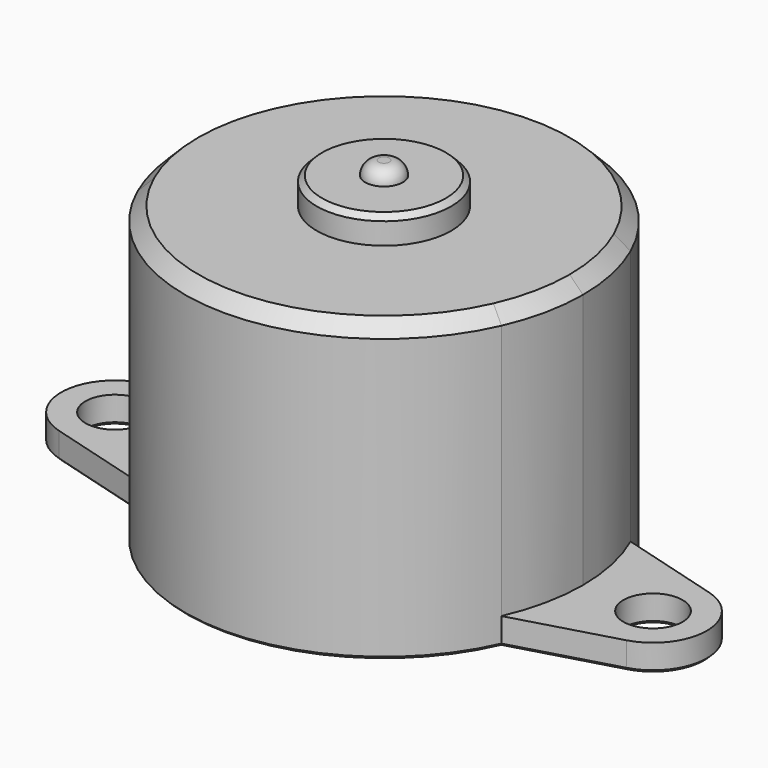
from build123d import *

# Parameters (mm, degrees)
F0_R     = 1.1
F1_DEPTH = 1
F3_DEPTH = 10
F4_R     = 2.5
F5_DEPTH = 1
F6_R     = 0.7
F7_DEPTH = 0.5
F8_R     = 0.49999
F9_SIZE  = 0.5
F10_SIZE = 0.1
F11_SIZE = 0.2


# Not quite as in the source:
# - a fillet or chamfer is up to 0.001 mm smaller than in the source, because OpenCascade refuses the exact size


with BuildPart() as f1:
    # F0 (on Top) → F1 (new body)
    with BuildSketch(Plane.XY):
        with BuildLine():
            ThreePointArc((-10.5473609378, 1.9236413397), (-12, 0), (-10.5473609378, -1.9236413397))
            Line((-10.5473609378, -1.9236413397), (-6.7646138101, -3))
            ThreePointArc((-6.7646138101, -3), (0, -7.4), (6.7646138101, -3))
            Line((6.7646138101, -3), (10.5473609378, -1.9236413397))
            ThreePointArc((10.5473609378, -1.9236413397), (12, 0), (10.5473609378, 1.9236413397))
            Line((10.5473609378, 1.9236413397), (6.7646138101, 3))
            ThreePointArc((6.7646138101, 3), (0, 7.4), (-6.7646138101, 3))
            Line((-6.7646138101, 3), (-10.5473609378, 1.9236413397))
        make_face()
        with Locations((-10, 0)):
            Circle(F0_R, mode=Mode.SUBTRACT)
        with Locations((10, 0)):
            Circle(F0_R, mode=Mode.SUBTRACT)
    extrude(amount=F1_DEPTH)

    # F2 (on face) → F3 (join)
    with BuildSketch(Plane.XY.offset(1)):
        with BuildLine():
            ThreePointArc((6.7646138101, -3), (7.2394109634, -1.5332739164), (7.4, 0))
            ThreePointArc((7.4, 0), (7.2394109634, 1.5332739164), (6.7646138101, 3))
            ThreePointArc((6.7646138101, 3), (0, 7.4), (-6.7646138101, 3))
            ThreePointArc((-6.7646138101, 3), (-7.4, 0), (-6.7646138101, -3))
            ThreePointArc((-6.7646138101, -3), (0, -7.4), (6.7646138101, -3))
        make_face()
    extrude(amount=F3_DEPTH)

    # F4 (on face) → F5 (join)
    with BuildSketch(Plane.XY.offset(11)):
        Circle(F4_R)
    extrude(amount=F5_DEPTH)

    # F6 (on face) → F7 (join)
    with BuildSketch(Plane.XY.offset(12)):
        Circle(F6_R)
    extrude(amount=F7_DEPTH)

    # F8 (radius 0.5 in the source; OpenCascade refuses exactly that, so slightly less here)
    f8_edges = [f1.edges().sort_by_distance(p)[0] for p in [
        (-0.7, 0, 12.5),
    ]]
    fillet(f8_edges, radius=F8_R)

    # F9
    f9_edges = [f1.edges().sort_by_distance(p)[0] for p in [
        (-7.4, 0, 11),
    ]]
    chamfer(f9_edges, length=F9_SIZE)

    # F10
    f10_edges = [f1.edges().sort_by_distance(p)[0] for p in [
        (-8.655987, 2.461821, 0),
        (-12, 0, 0),
        (-8.655987, -2.461821, 0),
        (0, -7.4, 0),
        (8.655987, -2.461821, 0),
        (12, 0, 0),
        (8.655987, 2.461821, 0),
        (0, 7.4, 0),
        (-11.1, 0, 0),
        (8.9, 0, 0),
    ]]
    chamfer(f10_edges, length=F10_SIZE)

    # F11
    f11_edges = [f1.edges().sort_by_distance(p)[0] for p in [
        (-2.5, 0, 12),
    ]]
    chamfer(f11_edges, length=F11_SIZE)


solid = f1.part
